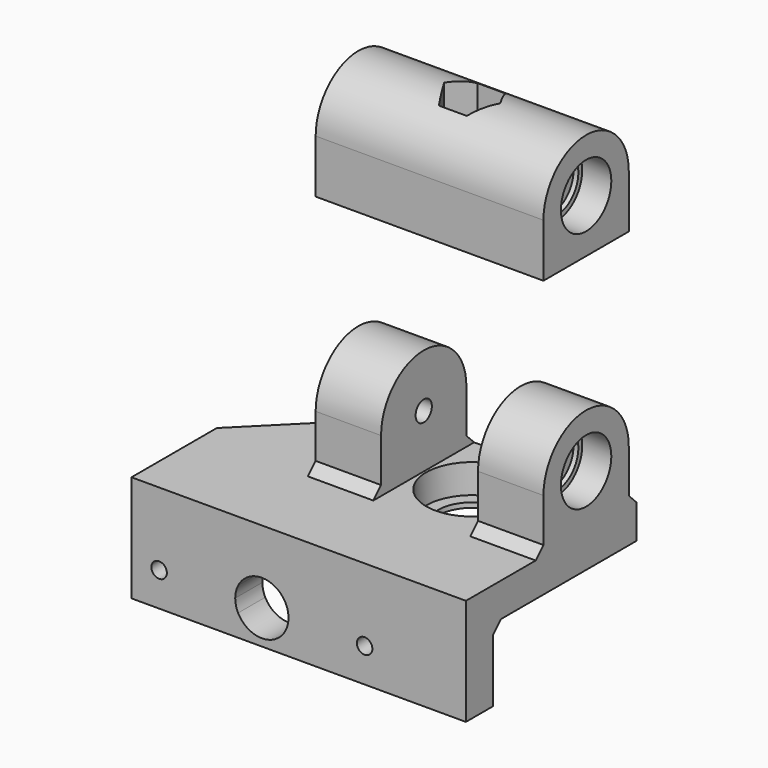
from build123d import *

# Parameters (mm, degrees)
F0_R      = 9.5
F1_DEPTH  = 7
F2_START  = -6
F0_R_2    = 7
F2_DEPTH  = 1
F3_W      = 47
F3_H      = 7
F4_DEPTH  = 14
F6_W      = 7
F6_H      = 14
F7_DEPTH  = 22
F9_START  = 10
F8_R      = 6.5
F9_DEPTH  = 13.5
F10_START = -10
F10_DEPTH = 13.5
F11_START = 10
F8_R_2    = 5.5
F11_DEPTH = 7.5
F12_START = -10
F12_DEPTH = 7.5
F13_START = -10
F8_R_3    = 2.1
F13_DEPTH = 6.5
F15_DEPTH = 22
F5_R      = 1.6
F5_R_2    = 4.85
F16_DEPTH = 25
F17_R     = 1.6
F18_DEPTH = 3
F19_DEPTH = 1
F20_SIZE  = 1.99999
F21_SIZE  = 22
F22_R     = 6.5
F23_DEPTH = 23.5
F22_R_2   = 5.5
F24_DEPTH = 17.5
F25_START = 10
F25_DEPTH = 6.5
F22_R_3   = 2.1
F26_DEPTH = 16.5
F28_START = -3
F27_R     = 3.5
F28_DEPTH = 22
F29_DEPTH = 25


# Not quite as in the source:
# - a fillet or chamfer is up to 0.001 mm smaller than in the source, because OpenCascade refuses the exact size


with BuildPart() as f1:
    # F0 (on Top) → F1 (new body)
    with BuildSketch(Plane.XY):
        Polygon((-23.5, 13), (-23.5, 0), (-23.5, -31), (23.5, -31), (23.5, 0), (23.5, 13), align=None)
        Circle(F0_R, mode=Mode.SUBTRACT)
    extrude(amount=-F1_DEPTH)

    # F0 (on Top) → F2 (join)
    with BuildSketch(Plane.XY.offset(F2_START)):
        Circle(F0_R)
        Circle(F0_R_2, mode=Mode.SUBTRACT)
    extrude(amount=-F2_DEPTH)

    # F3 (on face) → F4 (join)
    with BuildSketch(Plane(origin=(0, 0, -7), x_dir=(1, 0, 0), z_dir=(0, 0, -1))):
        with Locations((0, 27.5)):
            Rectangle(F3_W, F3_H)
    extrude(amount=F4_DEPTH)

    # F6 (on face) → F7 (join)
    with BuildSketch(Plane(origin=(-23.5, 0, 0), x_dir=(0, -1, 0), z_dir=(-1, 0, 0))):
        with Locations((27.5, -14)):
            Rectangle(F6_W, F6_H)
    extrude(amount=F7_DEPTH)

    # F8 (on Right) → F9 (join)
    with BuildSketch(Plane.YZ.offset(F9_START)):
        with BuildLine():
            Line((11, 0), (11, 11))
            ThreePointArc((11, 11), (7.7781745931, 3.2218254069), (0, 0))
            Line((0, 0), (11, 0))
        make_face()
        with BuildLine():
            ThreePointArc((0, 0), (-7.7781745931, 3.2218254069), (-11, 11))
            Line((-11, 11), (-11, 0))
            Line((-11, 0), (0, 0))
        make_face()
        with BuildLine():
            ThreePointArc((0, 0), (7.7781745931, 3.2218254069), (11, 11))
            ThreePointArc((11, 11), (0, 22), (-11, 11))
            ThreePointArc((-11, 11), (-7.7781745931, 3.2218254069), (0, 0))
        make_face()
        with Locations((0, 11)):
            Circle(F8_R, mode=Mode.SUBTRACT)
    extrude(amount=F9_DEPTH)

    # F8 (on Right) → F10 (join)
    with BuildSketch(Plane.YZ.offset(F10_START)):
        with BuildLine():
            ThreePointArc((0, 0), (-7.7781745931, 3.2218254069), (-11, 11))
            Line((-11, 11), (-11, 0))
            Line((-11, 0), (0, 0))
        make_face()
        with BuildLine():
            Line((11, 0), (11, 11))
            ThreePointArc((11, 11), (7.7781745931, 3.2218254069), (0, 0))
            Line((0, 0), (11, 0))
        make_face()
        with BuildLine():
            ThreePointArc((0, 0), (7.7781745931, 3.2218254069), (11, 11))
            ThreePointArc((11, 11), (0, 22), (-11, 11))
            ThreePointArc((-11, 11), (-7.7781745931, 3.2218254069), (0, 0))
        make_face()
        with Locations((0, 11)):
            Circle(F8_R, mode=Mode.SUBTRACT)
    extrude(amount=-F10_DEPTH)

    # F8 (on Right) → F11 (join)
    with BuildSketch(Plane.YZ.offset(F11_START)):
        with Locations((0, 11)):
            Circle(F8_R)
        with Locations((0, 11)):
            Circle(F8_R_2, mode=Mode.SUBTRACT)
    extrude(amount=F11_DEPTH)

    # F8 (on Right) → F12 (join)
    with BuildSketch(Plane.YZ.offset(F12_START)):
        with Locations((0, 11)):
            Circle(F8_R)
        with Locations((0, 11)):
            Circle(F8_R_2, mode=Mode.SUBTRACT)
    extrude(amount=-F12_DEPTH)

    # F8 (on Right) → F13 (join)
    with BuildSketch(Plane.YZ.offset(F13_START)):
        with Locations((0, 11)):
            Circle(F8_R_2)
        with Locations((0, 11)):
            Circle(F8_R_3, mode=Mode.SUBTRACT)
    extrude(amount=-F13_DEPTH)

    # F14 (on face) → F15 (join)
    with BuildSketch(Plane(origin=(-23.5, 0, 0), x_dir=(0, -1, 0), z_dir=(-1, 0, 0))):
        Polygon((-11, 0), (-13, 0), (-13, -7), (24, -7), (31, -7), (31, 0), (11, 0), align=None)
    extrude(amount=F15_DEPTH)

    # F5 (on face) → F16 (cut)
    with BuildSketch(Plane(origin=(0, -24, 0), x_dir=(-1, 0, 0), z_dir=(0, 1, 0))):
        with Locations((-2.6, -15)):
            Circle(F5_R)
        with Locations((39.8, -15)):
            Circle(F5_R)
        with BuildLine():
            Line((23.5, -17.4979991994), (23.5, -12.5020008006))
            ThreePointArc((23.5, -12.5020008006), (13.1, -15), (23.5, -17.4979991994))
        make_face()
        with Locations((18.6, -15)):
            Circle(F5_R_2, mode=Mode.SUBTRACT)
        with Locations((18.6, -15)):
            Circle(F5_R_2)
        with BuildLine():
            ThreePointArc((23.5, -17.4979991994), (23.9478967828, -16.2845232579), (24.1, -15))
            ThreePointArc((24.1, -15), (23.9478967828, -13.7154767421), (23.5, -12.5020008006))
            Line((23.5, -12.5020008006), (23.5, -17.4979991994))
        make_face()
    extrude(amount=-F16_DEPTH, mode=Mode.SUBTRACT)

    # F17 (on face) → F18 (cut)
    with BuildSketch(Plane(origin=(0, -24, 0), x_dir=(-1, 0, 0), z_dir=(0, 1, 0))):
        Polygon((-4.6207259422, -18.5), (-0.5792740578, -18.5), (1.4414518843, -15), (-0.5792740578, -11.5), (-4.6207259422, -11.5), (-6.6414518843, -15), align=None)
        with Locations((-2.6, -15)):
            Circle(F17_R, mode=Mode.SUBTRACT)
        Polygon((37.7792740578, -18.5), (41.8207259422, -18.5), (43.8414518843, -15), (41.8207259422, -11.5), (37.7792740578, -11.5), (35.7585481157, -15), align=None)
        with Locations((39.8, -15)):
            Circle(F17_R, mode=Mode.SUBTRACT)
    extrude(amount=-F18_DEPTH, mode=Mode.SUBTRACT)

    # F19 (add): a face of the model
    f19_faces = [f1.faces().sort_by_distance(p)[0] for p in [
        (-11, -27.5, -21),
    ]]
    extrude(f19_faces, amount=F19_DEPTH)

    # F20 (size 2 in the source; OpenCascade refuses exactly that, so slightly less here)
    f20_edges = [f1.edges().sort_by_distance(p)[0] for p in [
        (-11, -24, -7),
        (-16.75, 11, 0),
        (16.75, 11, 0),
        (16.75, -11, 0),
        (-16.75, -11, 0),
    ]]
    chamfer(f20_edges, length=F20_SIZE)

    # F21
    f21_edges = [f1.edges().sort_by_distance(p)[0] for p in [
        (-45.5, 13, -3.5),
    ]]
    chamfer(f21_edges, length=F21_SIZE)

    # F8 (on Right) → F25 (join)
    with BuildSketch(Plane.YZ.offset(F25_START)):
        with Locations((0, 11)):
            Circle(F8_R_2)
        with Locations((0, 11)):
            Circle(F8_R_3, mode=Mode.SUBTRACT)
    extrude(amount=F25_DEPTH)


with BuildPart() as f23:
    # F22 (on Right) → F23 (new body, symmetric)
    with BuildSketch(Plane.YZ):
        with BuildLine():
            ThreePointArc((0, 50), (7.7781745931, 53.2218254069), (11, 61))
            ThreePointArc((11, 61), (0, 72), (-11, 61))
            ThreePointArc((-11, 61), (-7.7781745931, 53.2218254069), (0, 50))
        make_face()
        with Locations((0, 61)):
            Circle(F22_R, mode=Mode.SUBTRACT)
        with BuildLine():
            ThreePointArc((0, 50), (-7.7781745931, 53.2218254069), (-11, 61))
            Line((-11, 61), (-11, 50))
            Line((-11, 50), (0, 50))
        make_face()
        with BuildLine():
            Line((11, 50), (11, 61))
            ThreePointArc((11, 61), (7.7781745931, 53.2218254069), (0, 50))
            Line((0, 50), (11, 50))
        make_face()
    extrude(amount=F23_DEPTH, both=True)

    # F22 (on Right) → F24 (join, symmetric)
    with BuildSketch(Plane.YZ):
        with Locations((0, 61)):
            Circle(F22_R)
        with Locations((0, 61)):
            Circle(F22_R_2, mode=Mode.SUBTRACT)
    extrude(amount=F24_DEPTH, both=True)

    # F22 (on Right) → F26 (join, symmetric)
    with BuildSketch(Plane.YZ):
        with Locations((0, 61)):
            Circle(F22_R_2)
        with Locations((0, 61)):
            Circle(F22_R_3, mode=Mode.SUBTRACT)
    extrude(amount=F26_DEPTH, both=True)

    # F27 (on face) → F28 (cut)
    with BuildSketch(Plane(origin=(0, 0, 50), x_dir=(1, 0, 0), z_dir=(0, 0, -1)).offset(F28_START)):
        Polygon((-2.8867513459, -5), (2.8867513459, -5), (5.7735026919, 0), (2.8867513459, 5), (-2.8867513459, 5), (-5.7735026919, 0), align=None)
        Circle(F27_R, mode=Mode.SUBTRACT)
        Circle(F27_R)
    extrude(amount=-F28_DEPTH, mode=Mode.SUBTRACT)

    # F27 (on face) → F29 (cut)
    with BuildSketch(Plane(origin=(0, 0, 50), x_dir=(1, 0, 0), z_dir=(0, 0, -1))):
        Circle(F27_R)
    extrude(amount=-F29_DEPTH, mode=Mode.SUBTRACT)


solid = Compound([f1.part, f23.part])
